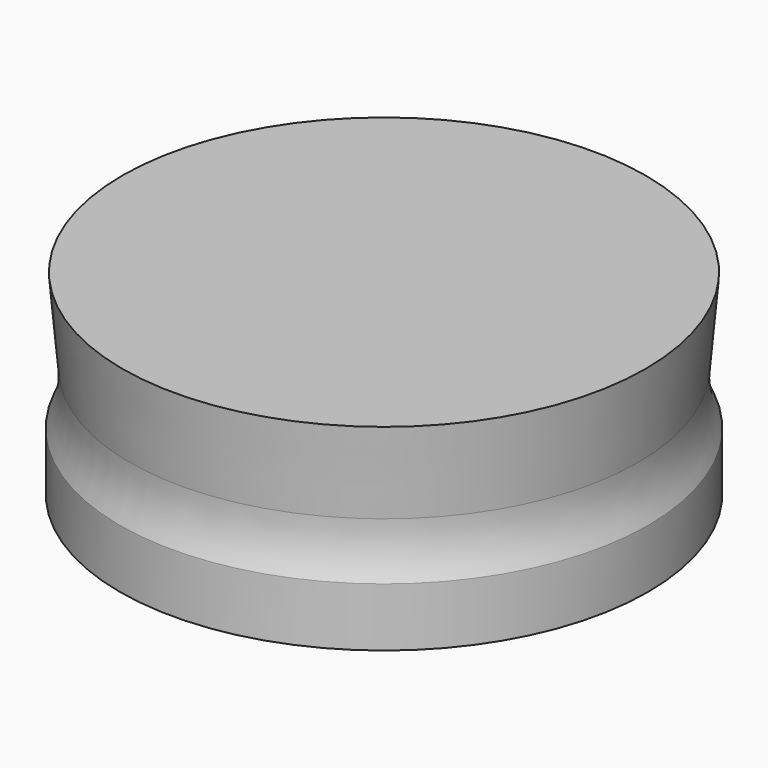
from build123d import *

# Parameters (mm, degrees)
F0_R     = 12.5
F1_DEPTH = 10
F1_TAPER = -5
F2_R     = 13.5
F3_DEPTH = 3


# Not quite as in the source:
# - a fillet or chamfer that OpenCascade refuses, or shapes differently, is made with other operations: its cross-section is extruded or revolved along the edge and cut away or added


with BuildPart() as f1:
    # F0 (on Top) → F1 (new body)
    with BuildSketch(Plane.XY):
        Circle(F0_R)
    extrude(amount=F1_DEPTH, taper=F1_TAPER)

    # F2 (on face) → F3 (join)
    with BuildSketch(Plane(origin=(0, 0, 0), x_dir=(1, 0, 0), z_dir=(0, 0, -1))):
        Circle(F2_R)
    extrude(amount=-F3_DEPTH)

    # F4: fillet of radius 5 on 1 edges, made by hand

    # F4_s1 → F4_t2 (revolve)
    with BuildSketch(Plane.XZ):
        with BuildLine():
            ThreePointArc((13.5, 3), (13.0638190953, 4.2967665116), (12.9954672306, 5.6632163606))
            Line((12.9954672306, 5.6632163606), (12.8958477608, 5.6719319348))
            Line((12.8958477608, 5.6719319348), (12.6628465208, 3.0087155743))
            Line((12.6628465208, 3.0087155743), (12.7624659906, 2.9))
            ThreePointArc((12.7624659906, 2.9), (13.1312329953, 2.9), (13.4104711856, 2.9554512471))
            Line((13.4104711856, 2.9554512471), (13.5, 3))
        make_face()
    revolve(axis=Axis((0, 0, 3), (0, 0, 1)))


solid = f1.part
